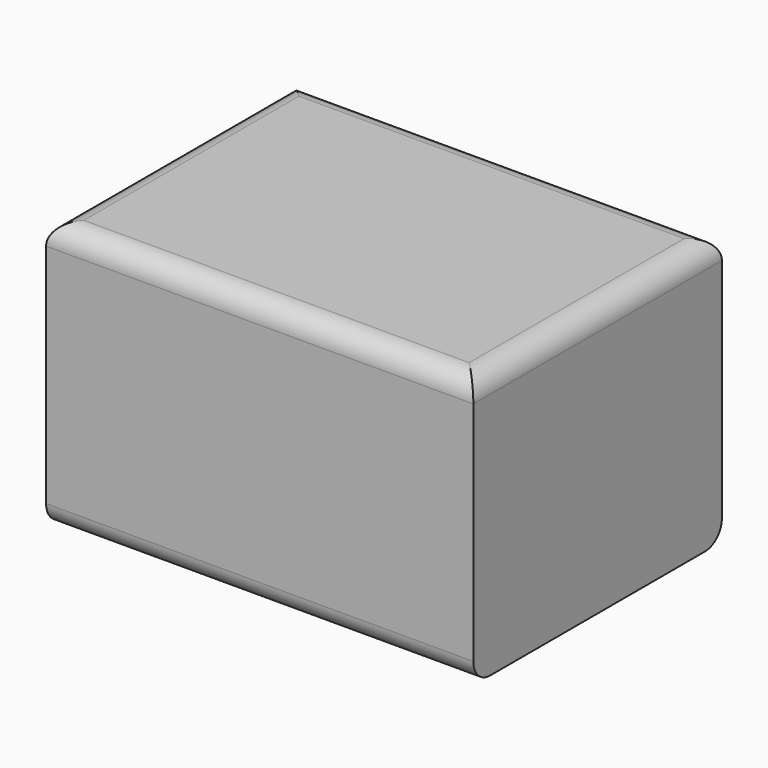
from build123d import *

# Parameters (mm, degrees)
F0_W        = 103.4230701625
F0_H        = 75.2167738974
F1_DEPTH    = 65.024
F2_T        = -2.54
F3_T1_DEPTH = 128.8230701625
F3_T3_DEPTH = 100.6167738974
F4_W        = 31.4045592836
F4_H        = 70.1367738974
F5_DEPTH    = 61.214
F6_R        = 15.24
F7_DEPTH    = 49.022


# Not quite as in the source:
# - a fillet or chamfer that OpenCascade refuses, or shapes differently, is made with other operations: its cross-section is extruded or revolved along the edge and cut away or added


with BuildPart() as f1:
    # F0 (on Top) → F1 (new body)
    with BuildSketch(Plane.XY):
        with Locations((6.9133061916, -6.8211276084)):
            Rectangle(F0_W, F0_H)
    extrude(amount=F1_DEPTH)

    # F2
    f2_openings = [f1.faces().sort_by_distance(p)[0] for p in [
        (6.913306, -6.821128, 0),
    ]]
    offset(amount=F2_T, openings=f2_openings)

    # F3: fillet of radius 5.08 on 6 edges, made by hand

    # F3_s2 → F3_t1 (cut)
    with BuildSketch(Plane.YZ.offset(-57.4982288897)):
        with BuildLine():
            ThreePointArc((-44.4295145571, 59.944), (-42.9416170056, 63.5361024484), (-39.3495145571, 65.024))
            Line((-39.3495145571, 65.024), (-44.4295145571, 65.024))
            Line((-44.4295145571, 65.024), (-44.4295145571, 59.944))
        make_face()
        with BuildLine():
            ThreePointArc((30.7872593403, 59.944), (29.2993617887, 63.5361024484), (25.7072593403, 65.024))
            Line((25.7072593403, 65.024), (30.7872593403, 65.024))
            Line((30.7872593403, 65.024), (30.7872593403, 59.944))
        make_face()
        with BuildLine():
            ThreePointArc((30.7872593403, 5.08), (29.2993617887, 1.4878975516), (25.7072593403, 0))
            Line((25.7072593403, 0), (30.7872593403, 0))
            Line((30.7872593403, 0), (30.7872593403, 5.08))
        make_face()
        with BuildLine():
            ThreePointArc((-44.4295145571, 5.08), (-42.9416170056, 1.4878975516), (-39.3495145571, 0))
            Line((-39.3495145571, 0), (-44.4295145571, 0))
            Line((-44.4295145571, 0), (-44.4295145571, 5.08))
        make_face()
    extrude(amount=F3_T1_DEPTH, mode=Mode.SUBTRACT)

    # F3_s4 → F3_t3 (cut)
    with BuildSketch(Plane.XZ.offset(-43.4872593403)):
        with BuildLine():
            ThreePointArc((-44.7982288897, 59.944), (-43.3103313381, 63.5361024484), (-39.7182288897, 65.024))
            Line((-39.7182288897, 65.024), (-44.7982288897, 65.024))
            Line((-44.7982288897, 65.024), (-44.7982288897, 59.944))
        make_face()
        with BuildLine():
            ThreePointArc((58.6248412728, 59.944), (57.1369437213, 63.5361024484), (53.5448412728, 65.024))
            Line((53.5448412728, 65.024), (58.6248412728, 65.024))
            Line((58.6248412728, 65.024), (58.6248412728, 59.944))
        make_face()
    extrude(amount=F3_T3_DEPTH, mode=Mode.SUBTRACT)

    # F4 (on face) → F5 (join)
    with BuildSketch(Plane(origin=(0, 0, 62.484), x_dir=(1, 0, 0), z_dir=(0, 0, -1))):
        Polygon((24.3728496134, 41.8895145571), (-10.8536696061, 41.8895145571), (-10.8536696061, -28.2472593403), (56.0848412728, -28.2472593403), (56.0848412728, 41.8895145571), align=None)
        with Locations((-26.5559492479, 6.8211276084)):
            Rectangle(F4_W, F4_H)
    extrude(amount=F5_DEPTH)

    # F6 (on face) → F7 (cut)
    with BuildSketch(Plane(origin=(0, 0, 1.27), x_dir=(1, 0, 0), z_dir=(0, 0, -1))):
        with Locations((-15.0351587272, 13.1098517179)):
            Circle(F6_R)
        with Locations((28.1448412728, 13.1098517179)):
            Circle(F6_R)
        with Locations((7.1306948804, -12.0557340983)):
            Circle(F6_R)
    extrude(amount=-F7_DEPTH, mode=Mode.SUBTRACT)


solid = f1.part
